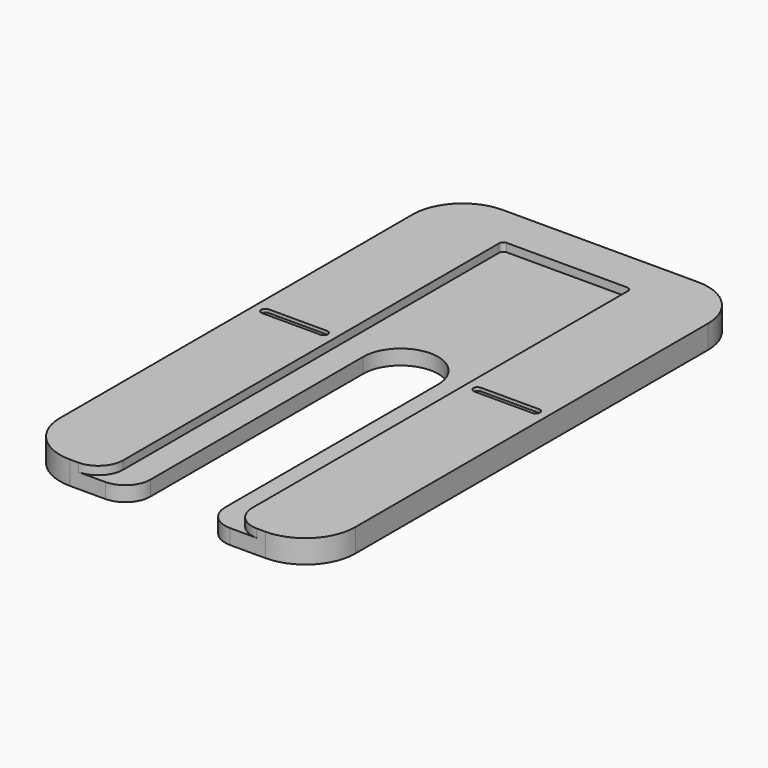
from build123d import *

# Parameters (mm, degrees)
F3_DEPTH = 2.8
F4_W     = 15.5
F4_H     = 60
F5_DEPTH = 25
F7_DEPTH = 0.4
F8_R     = 6
F9_R     = 0.5
F10_R    = 3


# Not quite as in the source:
# - a pattern or mirror of a feature is missing from the dataset's text; its kind, count and spacing are read off the source's solid


with BuildPart() as f3:
    # F2 (on Top) → F3 (new body)
    with BuildSketch(Plane.XY):
        with BuildLine():
            Line((4.5, -32.5), (17.75, -32.5))
            Line((17.75, -32.5), (17.75, 32.5))
            Line((17.75, 32.5), (-17.75, 32.5))
            Line((-17.75, 32.5), (-17.75, -32.5))
            Line((-17.75, -32.5), (-4.5, -32.5))
            Line((-4.5, -32.5), (-4.5, 2.5))
            ThreePointArc((-4.5, 2.5), (0, 7), (4.5, 2.5))
            Line((4.5, 2.5), (4.5, -32.5))
        make_face()
    extrude(amount=F3_DEPTH)

    # F4 (on offset) → F5 (cut)
    with BuildSketch(Plane.XY.offset(1.8)):
        with Locations((0, -2.5)):
            Rectangle(F4_W, F4_H)
    extrude(amount=F5_DEPTH, mode=Mode.SUBTRACT)

    # F6 (on face) → F7 (cut)
    with BuildSketch(Plane.XY.offset(2.8)):
        with BuildLine():
            Line((9.25, 2), (16.25, 2))
            ThreePointArc((16.25, 2), (16.75, 2.5), (16.25, 3))
            Line((16.25, 3), (9.25, 3))
            ThreePointArc((9.25, 3), (8.75, 2.5), (9.25, 2))
        make_face()
    f7 = extrude(amount=-F7_DEPTH, mode=Mode.SUBTRACT)

    # F7_copies: F7 across plane
    add(f7.mirror(Plane(origin=(0, 0, 0), x_dir=(0, 0, -1), z_dir=(-1, 0, 0))), mode=Mode.SUBTRACT)

    # F8
    f8_edges = [f3.edges().sort_by_distance(p)[0] for p in [
        (-17.75, -32.5, 1.4),
        (17.75, -32.5, 1.4),
        (-17.75, 32.5, 1.4),
        (17.75, 32.5, 1.4),
    ]]
    fillet(f8_edges, radius=F8_R)

    # F9
    f9_edges = [f3.edges().sort_by_distance(p)[0] for p in [
        (7.75, 27.5, 2.3),
        (-7.75, 27.5, 2.3),
    ]]
    fillet(f9_edges, radius=F9_R)

    # F10
    f10_edges = [f3.edges().sort_by_distance(p)[0] for p in [
        (7.75, -32.5, 2.3),
        (-7.75, -32.5, 2.3),
        (-4.5, -32.5, 0.9),
        (4.5, -32.5, 0.9),
    ]]
    fillet(f10_edges, radius=F10_R)


solid = f3.part
